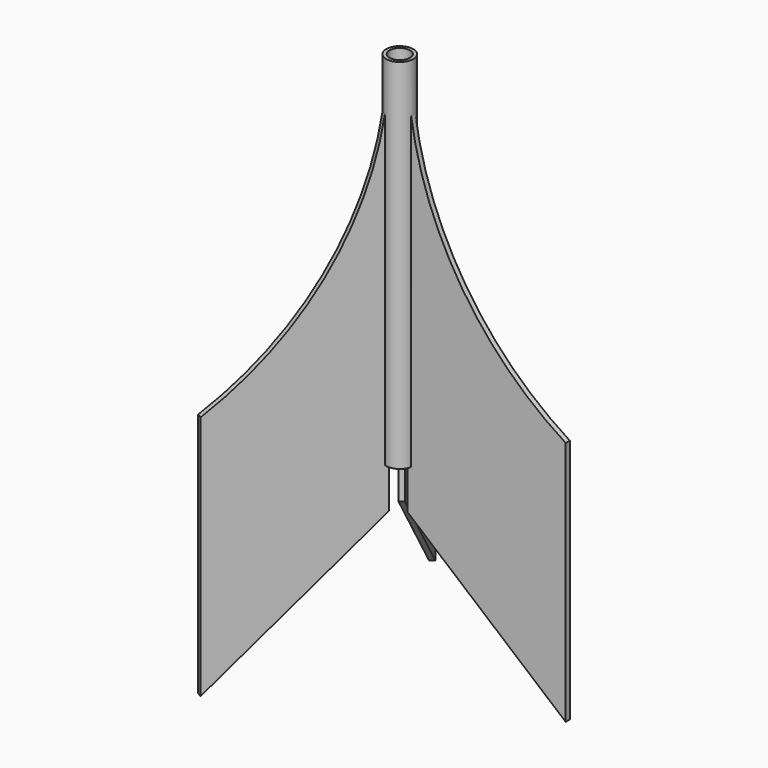
from build123d import *

# Parameters (mm, degrees)
F0_R          = 4.191
F0_R_2        = 2.921
F1_DEPTH      = 111.125
F3_DEPTH      = 0.79375
F3_DEPTH_BACK = 0.79375
F4_COUNT      = 3
F5_D          = 6.35
F5_DEPTH      = 111.1260001


# Not quite as in the source:
# - a length typed as a fraction of an inch, garbled in the dataset ("3 / 203.2 mm" for 3/8 in), is restored


with BuildPart() as f1:
    # F0 (on Top) → F1 (new body)
    with BuildSketch(Plane.XY):
        Circle(F0_R)
        Circle(F0_R_2, mode=Mode.SUBTRACT)
    extrude(amount=F1_DEPTH)

    # F2 (on Front) → F3 (join, two sides)
    with BuildSketch(Plane.XZ) as f3_sk:
        with BuildLine():
            ThreePointArc((52.1055692807, 22.1924969852), (16.1288428569, 60.3431066176), (3.05240741, 111.125))
            Line((3.05240741, 111.125), (3.05240741, -12.6199012697))
            Line((3.05240741, -12.6199012697), (52.1055692807, -12.6199012697))
            Line((52.1055692807, -12.6199012697), (52.1055692807, 22.1924969852))
        make_face()
        Polygon((52.1055692807, -12.6199012697), (3.05240741, -12.6199012697), (52.1055692807, -53.9700498879), align=None)
    extrude(amount=F3_DEPTH)
    extrude(f3_sk.sketch, amount=-F3_DEPTH_BACK)

    # F4: F1 ×3 about axis
    f4_axis = Axis((0, 0, 24.9059423804), (0, 0, -1))


with BuildPart() as f1_1:
    add(f1.part)
    for i in range(1, F4_COUNT):
        add(f1.part.rotate(f4_axis, i * 360 / F4_COUNT))

    # F5 (through all, one way)
    with BuildSketch(Plane(origin=(0, 0, 0), x_dir=(1, 0, 0), z_dir=(0, 0, -1))):
        with Locations((0, 0)):
            Circle(F5_D / 2)
    extrude(amount=-F5_DEPTH, mode=Mode.SUBTRACT)


solid = f1_1.part
